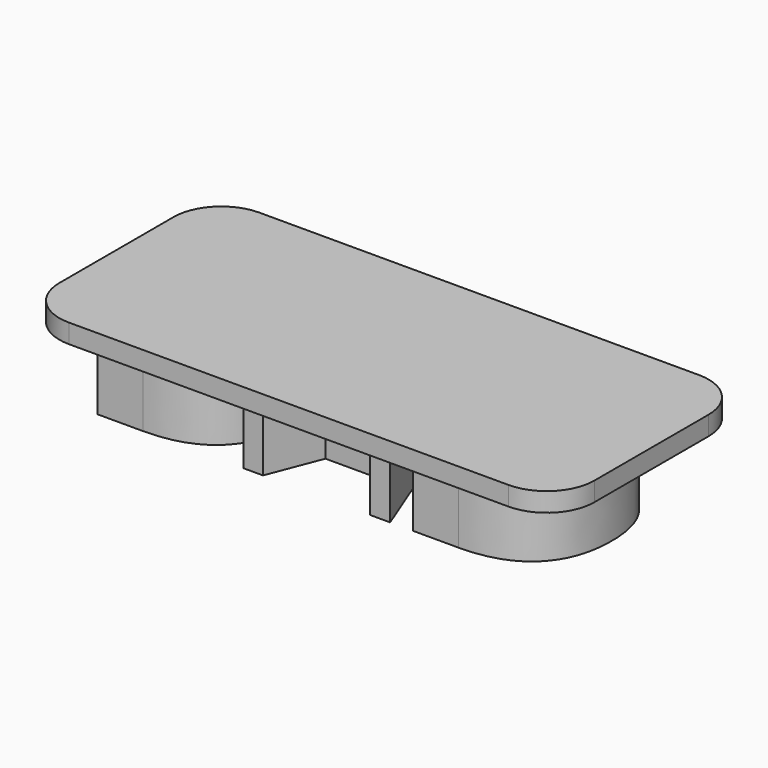
from build123d import *

# Parameters (mm, degrees)
F0_TEXT_SIZE = 30.8912396275
F1_DEPTH     = 10.16
F2_W         = 71.3450877304
F2_H         = 31.75
F3_DEPTH     = 2.54
F4_R         = 6.35


# Not quite as in the source:
# - Text() gives the source's letters only with a copy of the font that has no kerning and outlines rounded to 1/6400 em; it was checked with that copy


with BuildPart() as f1:
    # F0 (on Top) → F1 (new body)
    with BuildSketch(Plane.XY):
        with Locations((-32.3537467537, -11.1252)):
            Text('DAD', F0_TEXT_SIZE, font='Open Sans', text_align=(TextAlign.LEFT, TextAlign.BOTTOM))
    extrude(amount=-F1_DEPTH)


with BuildPart() as f3:
    # F2 (on Top) → F3 (new body)
    with BuildSketch(Plane.XY):
        Rectangle(F2_W, F2_H)
    extrude(amount=F3_DEPTH)

    # F4
    f4_edges = [f3.edges().sort_by_distance(p)[0] for p in [
        (-35.672544, 15.875, 1.27),
        (-35.672544, -15.875, 1.27),
        (35.672544, -15.875, 1.27),
        (35.672544, 15.875, 1.27),
    ]]
    fillet(f4_edges, radius=F4_R)


solid = Compound([f1.part, f3.part])
